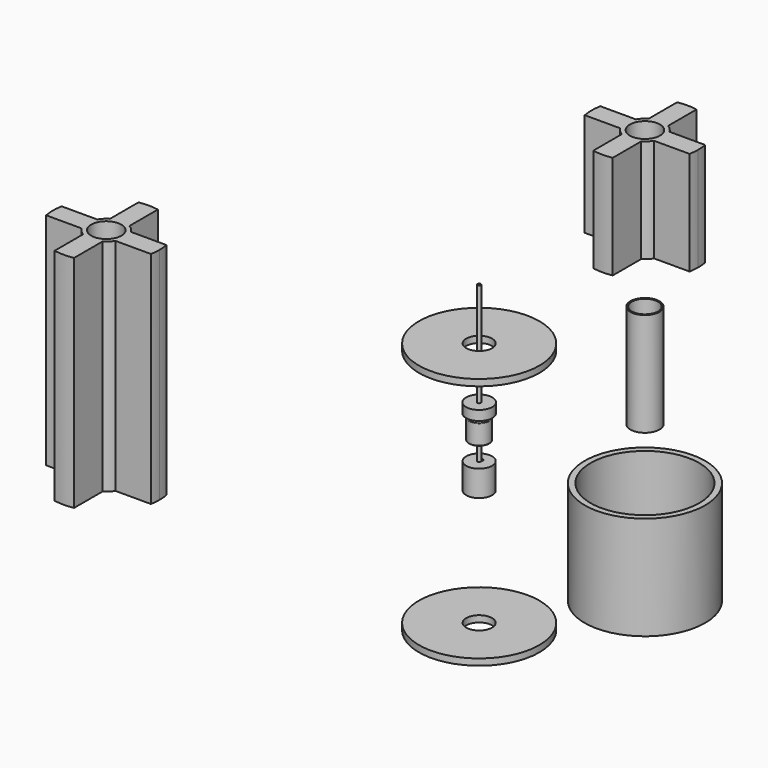
from build123d import *

# Parameters (mm, degrees)
F2_R      = 14.7701
F2_R_2    = 13.3223
F3_DEPTH  = 25.4
F5_R      = 3.571875
F5_R_2    = 3.216275
F6_DEPTH  = 25.4
F9_R      = 3.216275
F9_R_2    = 0.43815
F10_DEPTH = 2.38125
F12_R     = 3.698875
F13_DEPTH = 25.4
F15_R     = 2.5
F15_R_2   = 1
F16_DEPTH = 5
F17_R     = 0.15
F18_R     = 0.15
F21_R     = 3.175
F22_DEPTH = 6.35
F24_D     = 0.8382
F24_DEPTH = 0.8382
F24_TIP   = 0.2518206854
F25_R     = 0.4064
F27_DEPTH = 38.1
F28_R     = 14.7701
F28_R_2   = 3.175
F29_DEPTH = 1.5748
F31_R     = 14.7701
F31_R_2   = 3.175
F32_DEPTH = 1.5875
F34_R     = 3.698875
F35_DEPTH = 53.975


# Not quite as in the source:
# - a length typed as a fraction of an inch, garbled in the dataset ("3 / 203.2 mm" for 3/8 in), is restored
# - a feature names something its author has since deleted; it is built from what else it names


with BuildPart() as f3:
    # F2 (on Top) → F3 (new body)
    with BuildSketch(Plane.XY):
        Circle(F2_R)
        Circle(F2_R_2, mode=Mode.SUBTRACT)
    extrude(amount=-F3_DEPTH)


with BuildPart() as f3_1:
    # F4: moved
    add(f3.part.moved(Location((0, 50.8, -25.4))))


with BuildPart() as f6:
    # F5 (on Top) → F6 (new body)
    with BuildSketch(Plane.XY):
        Circle(F5_R)
        Circle(F5_R_2, mode=Mode.SUBTRACT)
    extrude(amount=-F6_DEPTH)


with BuildPart() as f6_1:
    # F7: moved
    add(f6.part.moved(Location((0, 50.8, 12.7))))


with BuildPart() as f10:
    # F9 (on Top) → F10 (new body)
    with BuildSketch(Plane.XY):
        Circle(F9_R)
        Circle(F9_R_2, mode=Mode.SUBTRACT)
    extrude(amount=-F10_DEPTH)


with BuildPart() as f10_1:
    # F11: moved
    add(f10.part.moved(Location((0, 0, 12.7))))


with BuildPart() as f13:
    # F12 (on Top) → F13 (new body)
    with BuildSketch(Plane.XY):
        with BuildLine():
            Line((2.38125, -12.8495180193), (2.38125, -4.1244459855))
            ThreePointArc((2.38125, -4.1244459855), (0, -4.7625), (-2.38125, -4.1244459855))
            Line((-2.38125, -4.1244459855), (-2.38125, -12.8495180193))
            ThreePointArc((-2.38125, -12.8495180193), (0, -13.0683), (2.38125, -12.8495180193))
        make_face()
        with BuildLine():
            ThreePointArc((-4.1244459855, -2.38125), (-4.7625, 0), (-4.1244459855, 2.38125))
            Line((-4.1244459855, 2.38125), (-12.8495180193, 2.38125))
            ThreePointArc((-12.8495180193, 2.38125), (-13.0683, 0), (-12.8495180193, -2.38125))
            Line((-12.8495180193, -2.38125), (-4.1244459855, -2.38125))
        make_face()
        with BuildLine():
            ThreePointArc((-2.38125, 4.1244459855), (0, 4.7625), (2.38125, 4.1244459855))
            Line((2.38125, 4.1244459855), (2.38125, 12.8495180193))
            ThreePointArc((2.38125, 12.8495180193), (0, 13.0683), (-2.38125, 12.8495180193))
            Line((-2.38125, 12.8495180193), (-2.38125, 4.1244459855))
        make_face()
        with BuildLine():
            ThreePointArc((4.1244459855, 2.38125), (4.6002217477, 1.2326257023), (4.7625, 0))
            ThreePointArc((4.7625, 0), (4.6002217477, -1.2326257023), (4.1244459855, -2.38125))
            Line((4.1244459855, -2.38125), (12.8495180193, -2.38125))
            ThreePointArc((12.8495180193, -2.38125), (13.0134895632, -1.1956396946), (13.0683, 0))
            ThreePointArc((13.0683, 0), (13.0134895632, 1.1956396946), (12.8495180193, 2.38125))
            Line((12.8495180193, 2.38125), (4.1244459855, 2.38125))
        make_face()
        with BuildLine():
            ThreePointArc((4.1244459855, -2.38125), (4.6002217477, -1.2326257023), (4.7625, 0))
            ThreePointArc((4.7625, 0), (4.6002217477, 1.2326257023), (4.1244459855, 2.38125))
            ThreePointArc((4.1244459855, 2.38125), (3.3675960454, 3.3675960454), (2.38125, 4.1244459855))
            ThreePointArc((2.38125, 4.1244459855), (0, 4.7625), (-2.38125, 4.1244459855))
            ThreePointArc((-2.38125, 4.1244459855), (-3.3675960454, 3.3675960454), (-4.1244459855, 2.38125))
            ThreePointArc((-4.1244459855, 2.38125), (-4.7625, 0), (-4.1244459855, -2.38125))
            ThreePointArc((-4.1244459855, -2.38125), (-3.3675960454, -3.3675960454), (-2.38125, -4.1244459855))
            ThreePointArc((-2.38125, -4.1244459855), (0, -4.7625), (2.38125, -4.1244459855))
            ThreePointArc((2.38125, -4.1244459855), (3.3675960454, -3.3675960454), (4.1244459855, -2.38125))
        make_face()
        Circle(F12_R, mode=Mode.SUBTRACT)
    extrude(amount=F13_DEPTH)


with BuildPart() as f13_1:
    # F14: moved
    add(f13.part.moved(Location((0, 50.8, 25.4))))


with BuildPart() as f16:
    # F15 (on Top) → F16 (new body)
    with BuildSketch(Plane.XY):
        Circle(F15_R)
        Circle(F15_R_2, mode=Mode.SUBTRACT)
    extrude(amount=-F16_DEPTH)

    # F17
    f17_edges = [f16.edges().sort_by_distance(p)[0] for p in [
        (-2.5, 0, -5),
    ]]
    fillet(f17_edges, radius=F17_R)

    # F18
    f18_edges = [f16.edges().sort_by_distance(p)[0] for p in [
        (-2.5, 0, 0),
    ]]
    fillet(f18_edges, radius=F18_R)


with BuildPart() as f16_1:
    # F19: moved
    add(f16.part.moved(Location((0, 0, 9.525))))


with BuildPart() as f22:
    # F21 (on Top) → F22 (new body)
    with BuildSketch(Plane.XY):
        Circle(F21_R)
    extrude(amount=-F22_DEPTH)

    # F24 (one way)
    with BuildSketch(Plane.XZ):
        with Locations((0, 0)):
            Circle(F24_D / 2)
    extrude(amount=-F24_DEPTH, mode=Mode.SUBTRACT)
    with Locations(Plane.XZ):
        with Locations((0, 0)):
            with Locations((0, 0, -(F24_DEPTH + F24_TIP / 2))):  # 118° drill point
                Cone(0, F24_D / 2, F24_TIP, mode=Mode.SUBTRACT)


with BuildPart() as f27:
    # F25 (on Top) → F27 (new body)
    with BuildSketch(Plane.XY):
        Circle(F25_R)
    extrude(amount=F27_DEPTH)


with BuildPart() as f29:
    # F28 (on Top) → F29 (new body)
    with BuildSketch(Plane.XY):
        Circle(F28_R)
        Circle(F28_R_2, mode=Mode.SUBTRACT)
    extrude(amount=-F29_DEPTH)


with BuildPart() as f29_1:
    # F30: moved
    add(f29.part.moved(Location((0, 0, -34.925))))


with BuildPart() as f32:
    # F31 (on Top) → F32 (new body)
    with BuildSketch(Plane.XY):
        Circle(F31_R)
        Circle(F31_R_2, mode=Mode.SUBTRACT)
    extrude(amount=-F32_DEPTH)


with BuildPart() as f32_1:
    # F33: moved
    add(f32.part.moved(Location((0, 0, 25.4))))


with BuildPart() as f35:
    # F34 (on Top) → F35 (new body)
    with BuildSketch(Plane.XY):
        with BuildLine():
            ThreePointArc((4.1244459855, -2.38125), (4.6002217477, -1.2326257023), (4.7625, 0))
            ThreePointArc((4.7625, 0), (4.6002217477, 1.2326257023), (4.1244459855, 2.38125))
            ThreePointArc((4.1244459855, 2.38125), (3.3675960454, 3.3675960454), (2.38125, 4.1244459855))
            ThreePointArc((2.38125, 4.1244459855), (0, 4.7625), (-2.38125, 4.1244459855))
            ThreePointArc((-2.38125, 4.1244459855), (-3.3675960454, 3.3675960454), (-4.1244459855, 2.38125))
            ThreePointArc((-4.1244459855, 2.38125), (-4.7625, 0), (-4.1244459855, -2.38125))
            ThreePointArc((-4.1244459855, -2.38125), (-3.3675960454, -3.3675960454), (-2.38125, -4.1244459855))
            ThreePointArc((-2.38125, -4.1244459855), (0, -4.7625), (2.38125, -4.1244459855))
            ThreePointArc((2.38125, -4.1244459855), (3.3675960454, -3.3675960454), (4.1244459855, -2.38125))
        make_face()
        Circle(F34_R, mode=Mode.SUBTRACT)
        with BuildLine():
            ThreePointArc((-2.38125, 4.1244459855), (0, 4.7625), (2.38125, 4.1244459855))
            Line((2.38125, 4.1244459855), (2.38125, 12.8495180193))
            ThreePointArc((2.38125, 12.8495180193), (0, 13.0683), (-2.38125, 12.8495180193))
            Line((-2.38125, 12.8495180193), (-2.38125, 4.1244459855))
        make_face()
        with BuildLine():
            ThreePointArc((4.1244459855, 2.38125), (4.6002217477, 1.2326257023), (4.7625, 0))
            ThreePointArc((4.7625, 0), (4.6002217477, -1.2326257023), (4.1244459855, -2.38125))
            Line((4.1244459855, -2.38125), (12.8495180193, -2.38125))
            ThreePointArc((12.8495180193, -2.38125), (13.0134895632, -1.1956396946), (13.0683, 0))
            ThreePointArc((13.0683, 0), (13.0134895632, 1.1956396946), (12.8495180193, 2.38125))
            Line((12.8495180193, 2.38125), (4.1244459855, 2.38125))
        make_face()
        with BuildLine():
            ThreePointArc((-4.1244459855, -2.38125), (-4.7625, 0), (-4.1244459855, 2.38125))
            Line((-4.1244459855, 2.38125), (-12.8495180193, 2.38125))
            ThreePointArc((-12.8495180193, 2.38125), (-13.0683, 0), (-12.8495180193, -2.38125))
            Line((-12.8495180193, -2.38125), (-4.1244459855, -2.38125))
        make_face()
        with BuildLine():
            Line((2.38125, -12.8495180193), (2.38125, -4.1244459855))
            ThreePointArc((2.38125, -4.1244459855), (0, -4.7625), (-2.38125, -4.1244459855))
            Line((-2.38125, -4.1244459855), (-2.38125, -12.8495180193))
            ThreePointArc((-2.38125, -12.8495180193), (0, -13.0683), (2.38125, -12.8495180193))
        make_face()
    extrude(amount=F35_DEPTH)


with BuildPart() as f35_1:
    # F36: moved
    add(f35.part.moved(Location((-50.8, -50.8, 0))))


solid = Compound([f3_1.part, f6_1.part, f10_1.part, f13_1.part, f16_1.part, f22.part, f27.part, f29_1.part, f32_1.part, f35_1.part])
